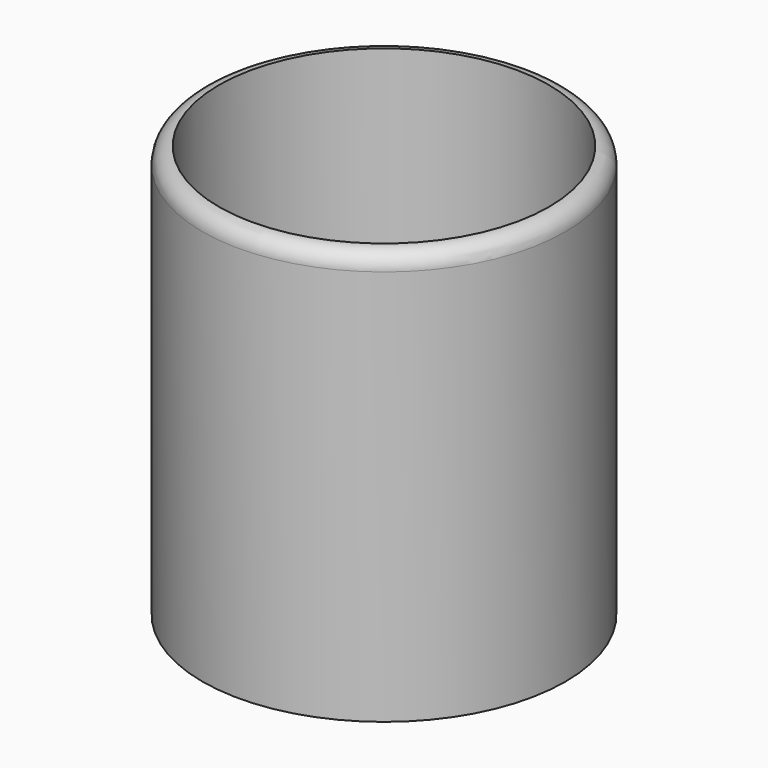
from build123d import *

# Parameters (mm, degrees)
F0_R     = 11
F1_DEPTH = 25
F2_R     = 10
F3_DEPTH = 22
F4_SIZE  = 0.5
F5_R     = 0.99999


# Not quite as in the source:
# - a fillet or chamfer is up to 0.001 mm smaller than in the source, because OpenCascade refuses the exact size


with BuildPart() as f1:
    # F0 (on Top) → F1 (new body)
    with BuildSketch(Plane.XY):
        Circle(F0_R)
    extrude(amount=F1_DEPTH)

    # F2 (on face) → F3 (cut)
    with BuildSketch(Plane.XY.offset(25)):
        Circle(F2_R)
    extrude(amount=-F3_DEPTH, mode=Mode.SUBTRACT)

    # F4
    f4_edges = [f1.edges().sort_by_distance(p)[0] for p in [
        (-10, 0, 3),
    ]]
    chamfer(f4_edges, length=F4_SIZE)

    # F5 (radius 1 in the source; OpenCascade refuses exactly that, so slightly less here)
    f5_edges = [f1.edges().sort_by_distance(p)[0] for p in [
        (-11, 0, 25),
    ]]
    fillet(f5_edges, radius=F5_R)


solid = f1.part
